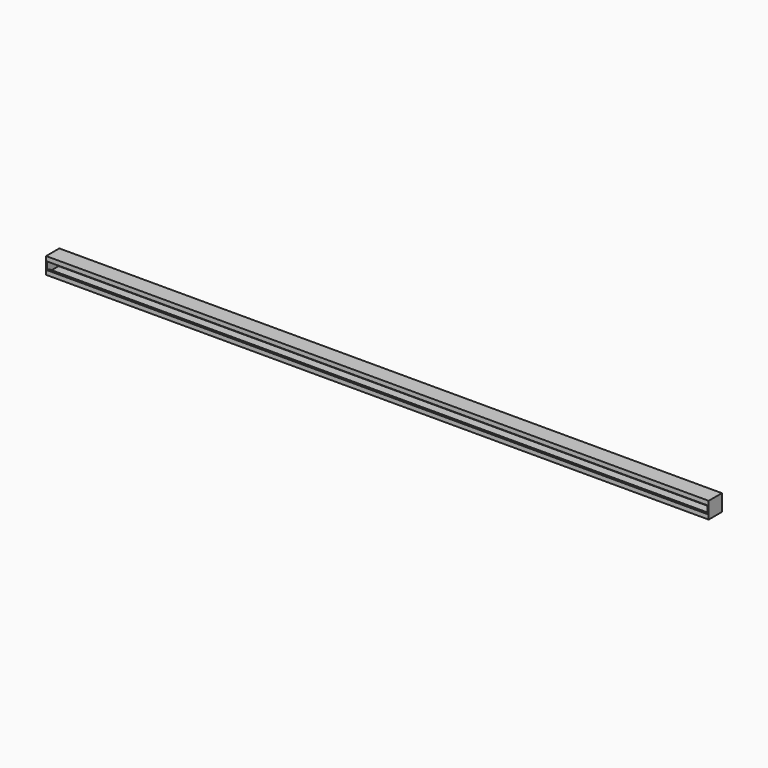
from build123d import *

# Parameters (mm, degrees)
F1_DEPTH = 299
F3_W     = 15
F3_H     = 15
F4_DEPTH = 1
F6_W     = 15
F6_H     = 15
F7_DEPTH = 1


# Not quite as in the source:
# - the program builds the solid bodies; features that only make, move or delete a surface that nothing else refers to are left out


with BuildPart() as f1:
    # F0 (on Right) → F1 (new body, symmetric)
    with BuildSketch(Plane.YZ):
        Polygon((7.5, 7.5), (-7.5, 7.5), (-7.5, 3.5), (-5.5, 3.5), (-5.5, 5.5), (5.5, 5.5), (5.5, -5.5), (-5.5, -5.5), (-5.5, -3.5), (-7.5, -3.5), (-7.5, -7.5), (7.5, -7.5), align=None)
    extrude(amount=F1_DEPTH, both=True)

    # F3 (on offset) → F4 (join)
    with BuildSketch(Plane.YZ.offset(299)):
        Rectangle(F3_W, F3_H)
    extrude(amount=F4_DEPTH)

    # F6 (on offset) → F7 (join)
    with BuildSketch(Plane(origin=(-299, 0, 0), x_dir=(0, -1, 0), z_dir=(-1, 0, 0))):
        Rectangle(F6_W, F6_H)
    extrude(amount=F7_DEPTH)


solid = f1.part
